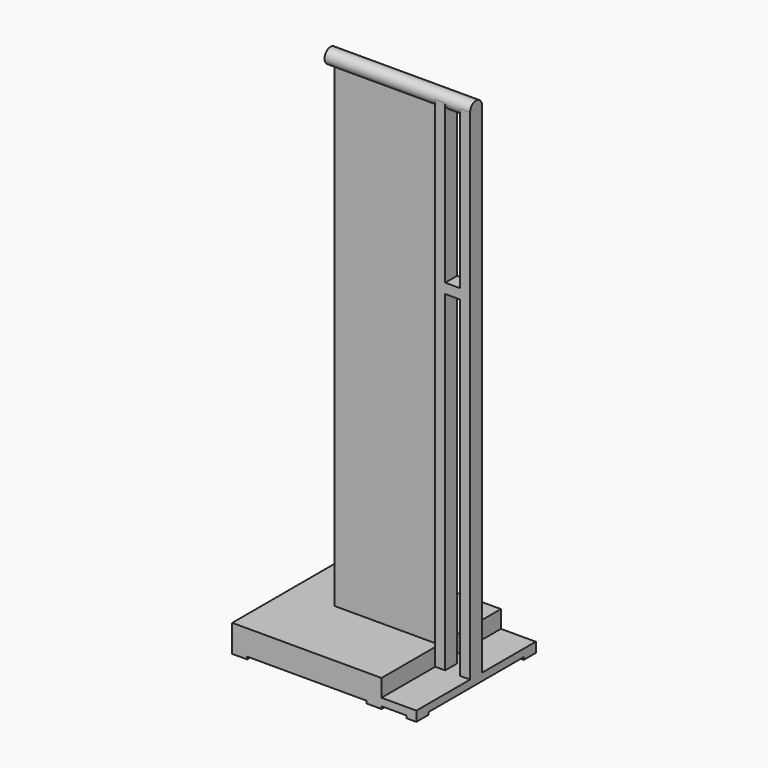
from build123d import *

# Parameters (mm, degrees)
F0_W           = 30
F0_H           = 30
F1_DEPTH       = 5.5
F2_T           = -1.5
F3_W           = 2
F3_H           = 102.35
F4_DEPTH       = 1.5
F6_DEPTH       = 29.25
F7_W           = 7
F7_H           = 30
F8_DEPTH       = 2
F10_W          = 24
F10_H          = 0.5
F10_W_2        = 5
F11_DEPTH      = 25
F12_W          = 3
F12_H          = 2
F13_DEPTH      = 1.5
F13_DEPTH_BACK = 1.5
F14_W          = 21
F14_H          = 95.85
F15_DEPTH      = 0.5


# Not quite as in the source:
# - a pattern or mirror of a feature is missing from the dataset's text; its kind, count and spacing are read off the source's solid


with BuildPart() as f1:
    # F0 (on Top) → F1 (new body)
    with BuildSketch(Plane.XY):
        Rectangle(F0_W, F0_H)
    extrude(amount=F1_DEPTH)

    # F2
    f2_openings = [f1.faces().sort_by_distance(p)[0] for p in [
        (0, 0, 0),
    ]]
    offset(amount=F2_T, openings=f2_openings)

    # F3 (on Front) → F4 (join, symmetric)
    with BuildSketch(Plane.XZ):
        with Locations((16, 51.175)):
            Rectangle(F3_W, F3_H)
    extrude(amount=F4_DEPTH, both=True)



with BuildPart() as f4:
    # F3 (on Front) → F4, piece 2 (new body, symmetric)
    with BuildSketch(Plane.XZ):
        with Locations((21, 51.175)):
            Rectangle(F3_W, F3_H)
    extrude(amount=F4_DEPTH, both=True)


with BuildPart() as f1_1:
    add(f1.part)

    add(f4.part)  # F6 merges F4
    # F5 (on face) → F6 (join)
    with BuildSketch(Plane.YZ.offset(22)):
        with BuildLine():
            ThreePointArc((-1.5, 102.35), (0, 100.85), (1.5, 102.35))
            Line((1.5, 102.35), (-1.5, 102.35))
        make_face()
        with BuildLine():
            Line((-1.5, 102.35), (1.5, 102.35))
            ThreePointArc((1.5, 102.35), (0, 103.85), (-1.5, 102.35))
        make_face()
    extrude(amount=-F6_DEPTH)

    # F7 (on Top) → F8 (join)
    with BuildSketch(Plane.XY):
        with Locations((18.5, 0)):
            Rectangle(F7_W, F7_H)
    extrude(amount=F8_DEPTH)

    # F10 (on Front) → F11 (cut, symmetric)
    with BuildSketch(Plane.XZ):
        with Locations((0, 0.25)):
            Rectangle(F10_W, F10_H)
        with Locations((17.5, 0.25)):
            Rectangle(F10_W_2, F10_H)
    f11 = extrude(amount=F11_DEPTH, both=True, mode=Mode.SUBTRACT)

    # F11_copies: F11 across plane
    add(f11.mirror(Plane(origin=(0, 0, 0), x_dir=(-0.7071067812, 0.7071067812, 0), z_dir=(-0.7071067812, -0.7071067812, 0))), mode=Mode.SUBTRACT)

    # F12 (on Front) → F13 (join, two sides)
    with BuildSketch(Plane.XZ) as f13_sk:
        with Locations((18.5, 69.6)):
            Rectangle(F12_W, F12_H)
    extrude(amount=F13_DEPTH)
    extrude(f13_sk.sketch, amount=-F13_DEPTH_BACK)

    # F14 (on Front) → F15 (join, symmetric)
    with BuildSketch(Plane.XZ):
        with Locations((4.5, 53.425)):
            Rectangle(F14_W, F14_H)
    extrude(amount=F15_DEPTH, both=True)


solid = f1_1.part
